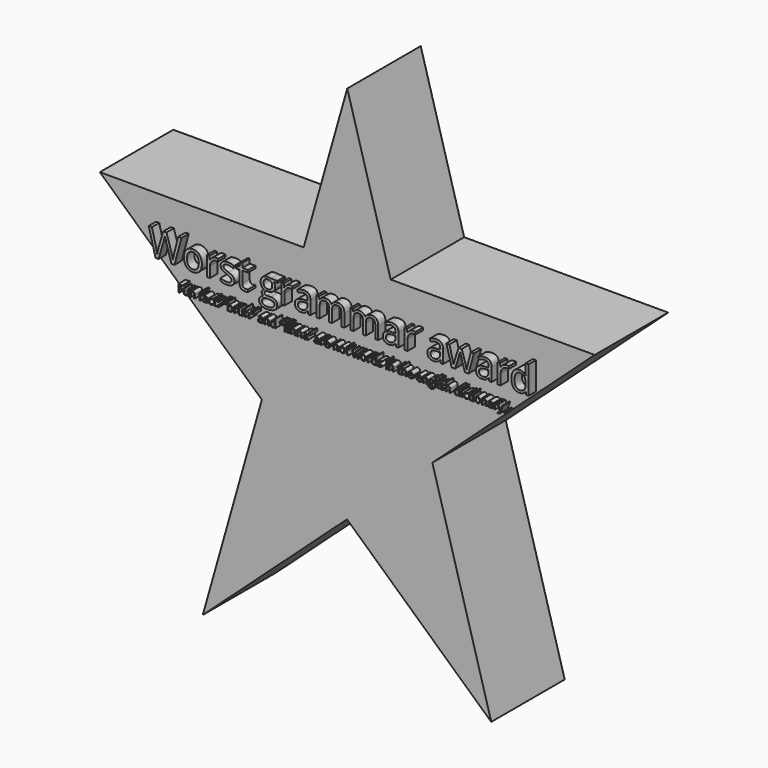
from build123d import *

# Parameters (mm, degrees)
F2_DEPTH       = 25.4
F3_TEXT_SIZE   = 10.0726715985
F3_TEXT_SIZE_2 = 2.9310948905
F4_DEPTH       = 2.54


# Not quite as in the source:
# - the program builds the solid bodies; features that only make, move or delete a surface that nothing else refers to are left out
# - Text() gives the source's letters only with a copy of the font that has no kerning and outlines rounded to 1/6400 em; it was checked with that copy


with BuildPart() as f2:
    # F0 (on Front) → F2 (new body)
    with BuildSketch(Plane.XZ):
        Polygon((-0.0800414132, -28.6863729593), (39.8404149541, -65.0694368672), (23.5353694415, -7.2138047278), align=None)
        Polygon((-23.6403090517, -7.2138047278), (-39.9917561256, -64.9765320706), (-0.0800414132, -28.6863729593), align=None)
        Polygon((-12.0728000112, 33.6492985635), (-68.4763826739, 33.6492985635), (-23.6403090517, -7.2138047278), align=None)
        Polygon((23.5353694415, -7.2138047278), (12.0192087098, 33.6492985635), (-12.0728000112, 33.6492985635), (-23.6403090517, -7.2138047278), (-0.0800414132, -28.6863729593), align=None)
        Polygon((12.0192087098, 33.6492985635), (0, 76.2973805443), (-12.0728000112, 33.6492985635), align=None)
        Polygon((23.5353694415, -7.2138047278), (68.4763826739, 33.6492985635), (12.0192087098, 33.6492985635), align=None)
    extrude(amount=F2_DEPTH)

    # F3 (on face) → F4 (join)
    with BuildSketch(Plane.XZ.offset(25.4)):
        with Locations((-53.0631070979, 19.4389195578)):
            Text('Worst grammar award', F3_TEXT_SIZE, font='Open Sans', text_align=(TextAlign.LEFT, TextAlign.BOTTOM))
        with Locations((-45.0216354831, 13.0785969917)):
            Text('Fun fact: "bruh" and "finna\' are not words in the english dictionary.', F3_TEXT_SIZE_2, font='Open Sans', text_align=(TextAlign.LEFT, TextAlign.BOTTOM))
    extrude(amount=F4_DEPTH)


solid = f2.part
